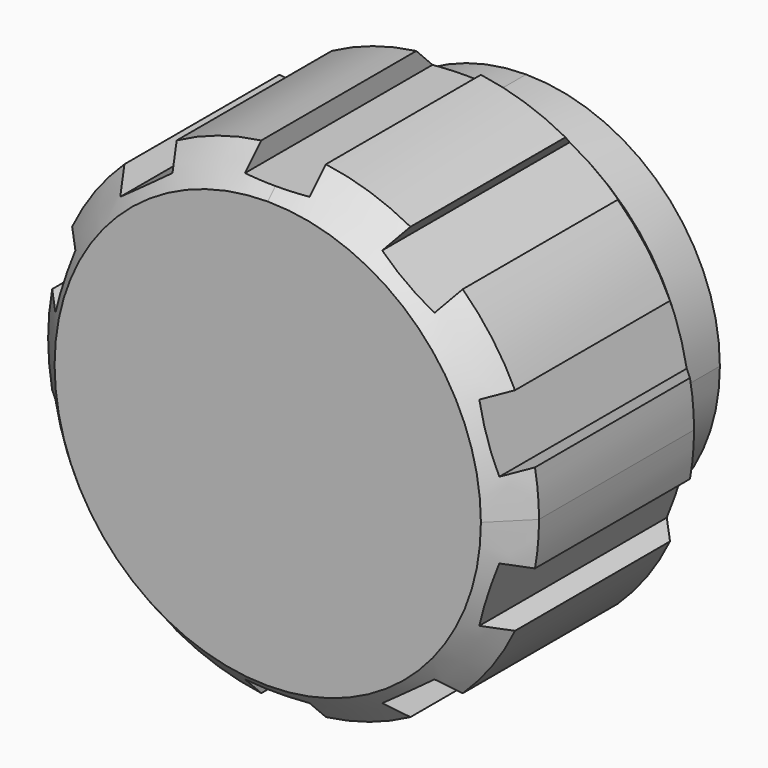
from build123d import *

# Parameters (mm, degrees)
F1_DEPTH = 1
F2_DEPTH = 4
F3_SIZE  = 0.5
F5_DEPTH = 10


# Not quite as in the source:
# - a feature names something its author has since deleted; it is built from what else it names


with BuildPart() as f1:
    # F0 (on Front) → F1 (new body)
    with BuildSketch(Plane.XZ):
        with BuildLine():
            ThreePointArc((3, 0), (2.1213203436, 2.1213203436), (0, 3))
            ThreePointArc((0, 3), (-2.1213203436, -2.1213203436), (3, 0))
        make_face()
    extrude(amount=-F1_DEPTH)

    # F0 (on Front) → F2 (join)
    with BuildSketch(Plane.XZ):
        with BuildLine():
            ThreePointArc((0, 3.8), (-2.6870057685, -2.6870057685), (3.8, 0))
            ThreePointArc((3.8, 0), (2.6870057685, 2.6870057685), (0, 3.8))
        make_face()
        with BuildLine():
            ThreePointArc((3, 0), (-2.1213203436, -2.1213203436), (0, 3))
            ThreePointArc((0, 3), (2.1213203436, 2.1213203436), (3, 0))
        make_face(mode=Mode.SUBTRACT)
        with BuildLine():
            ThreePointArc((3, 0), (2.1213203436, 2.1213203436), (0, 3))
            ThreePointArc((0, 3), (-2.1213203436, -2.1213203436), (3, 0))
        make_face()
    extrude(amount=F2_DEPTH)

    # F3
    f3_edges = [f1.edges().sort_by_distance(p)[0] for p in [
        (0, -4, -3.8),
        (0, 0, -3.8),
    ]]
    chamfer(f3_edges, length=F3_SIZE)

    # F4 (on face) → F5 (cut)
    with BuildSketch(Plane(origin=(0, 1, 0), x_dir=(-1, 0, 0), z_dir=(0, 1, 0))):
        with BuildLine():
            Line((-1.6233506232, 3.0850012567), (-1.809656001, 3.3414286104))
            ThreePointArc((-1.809656001, 3.3414286104), (-2.2335839587, 3.0742645786), (-2.6186729953, 2.7536433581))
            Line((-2.6186729953, 2.7536433581), (-2.4323676176, 2.4972160044))
            Line((-2.4323676176, 2.4972160044), (-1.6233506232, 3.0850012567))
        make_face()
        with BuildLine():
            Line((0, 3.45), (0, 3.8))
            ThreePointArc((0, 3.8), (-0.2505451722, 3.7917314141), (-0.5, 3.7669616404))
            Line((-0.5, 3.7669616404), (-0.5, 3.45))
            Line((-0.5, 3.45), (0, 3.45))
        make_face()
        with BuildLine():
            Line((0.5, 3.45), (0.5, 3.7669616404))
            ThreePointArc((0.5, 3.7669616404), (0.2505451722, 3.7917314141), (0, 3.8))
            Line((0, 3.8), (0, 3.45))
            Line((0, 3.45), (0.5, 3.45))
        make_face()
        with BuildLine():
            ThreePointArc((3.4280849175, -1.6395834222), (3.6140147619, -1.1742645786), (3.7371019119, -0.6885269059))
            Line((3.7371019119, -0.6885269059), (3.4356534784, -0.5905803724))
            Line((3.4356534784, -0.5905803724), (3.126636484, -1.5416368887))
            Line((3.126636484, -1.5416368887), (3.4280849175, -1.6395834222))
        make_face()
        with BuildLine():
            ThreePointArc((1.809656001, -3.3414286104), (2.2335839587, -3.0742645786), (2.6186729953, -2.7536433581))
            Line((2.6186729953, -2.7536433581), (2.4323676176, -2.4972160044))
            Line((2.4323676176, -2.4972160044), (1.6233506232, -3.0850012567))
            Line((1.6233506232, -3.0850012567), (1.809656001, -3.3414286104))
        make_face()
        with BuildLine():
            ThreePointArc((-0.5, -3.7669616404), (0, -3.8), (0.5, -3.7669616404))
            Line((0.5, -3.7669616404), (0.5, -3.45))
            Line((0.5, -3.45), (-0.5, -3.45))
            Line((-0.5, -3.45), (-0.5, -3.7669616404))
        make_face()
        with BuildLine():
            ThreePointArc((-2.6186729953, -2.7536433581), (-2.2335839587, -3.0742645786), (-1.809656001, -3.3414286104))
            Line((-1.809656001, -3.3414286104), (-1.6233506232, -3.0850012567))
            Line((-1.6233506232, -3.0850012567), (-2.4323676176, -2.4972160044))
            Line((-2.4323676176, -2.4972160044), (-2.6186729953, -2.7536433581))
        make_face()
        with BuildLine():
            ThreePointArc((-3.7371019119, -0.6885269059), (-3.6140147619, -1.1742645786), (-3.4280849175, -1.6395834222))
            Line((-3.4280849175, -1.6395834222), (-3.126636484, -1.5416368887))
            Line((-3.126636484, -1.5416368887), (-3.4356534784, -0.5905803724))
            Line((-3.4356534784, -0.5905803724), (-3.7371019119, -0.6885269059))
        make_face()
        with BuildLine():
            Line((-3.126636484, 1.5416368887), (-3.4280849175, 1.6395834222))
            ThreePointArc((-3.4280849175, 1.6395834222), (-3.6140147619, 1.1742645786), (-3.7371019119, 0.6885269059))
            Line((-3.7371019119, 0.6885269059), (-3.4356534784, 0.5905803724))
            Line((-3.4356534784, 0.5905803724), (-3.126636484, 1.5416368887))
        make_face()
        with BuildLine():
            Line((3.4356534784, 0.5905803724), (3.7371019119, 0.6885269059))
            ThreePointArc((3.7371019119, 0.6885269059), (3.6140147619, 1.1742645786), (3.4280849175, 1.6395834222))
            Line((3.4280849175, 1.6395834222), (3.126636484, 1.5416368887))
            Line((3.126636484, 1.5416368887), (3.4356534784, 0.5905803724))
        make_face()
        with BuildLine():
            Line((2.4323676176, 2.4972160044), (2.6186729953, 2.7536433581))
            ThreePointArc((2.6186729953, 2.7536433581), (2.2335839587, 3.0742645786), (1.809656001, 3.3414286104))
            Line((1.809656001, 3.3414286104), (1.6233506232, 3.0850012567))
            Line((1.6233506232, 3.0850012567), (2.4323676176, 2.4972160044))
        make_face()
    extrude(amount=-F5_DEPTH, mode=Mode.SUBTRACT)


solid = f1.part
